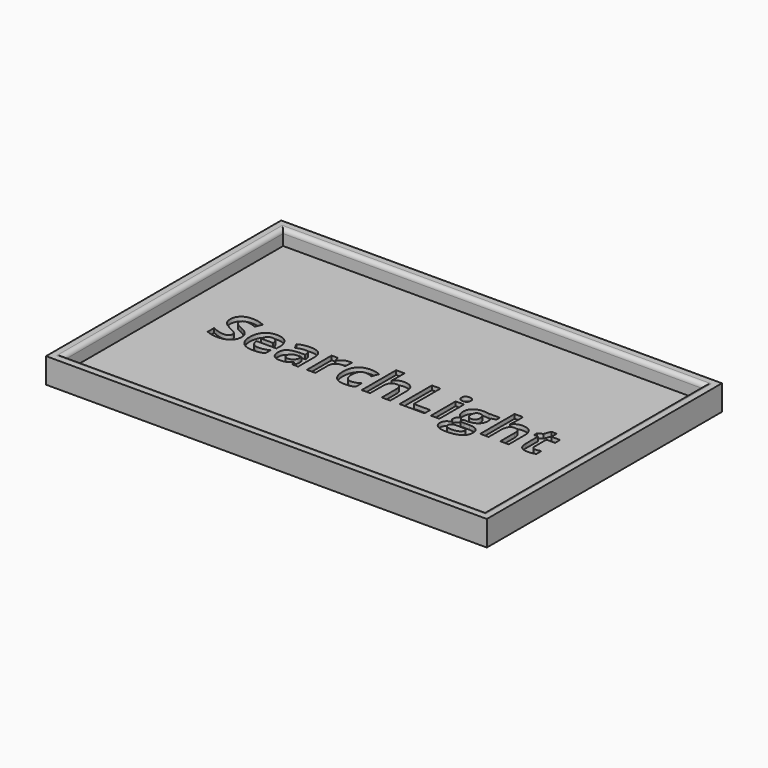
from build123d import *

# Parameters (mm, degrees)
F0_W         = 105
F0_H         = 70
F1_DEPTH     = 6
F2_T         = -2.4
F3_T1_DEPTH  = 65.2
F3_T3_DEPTH  = 100.2
F3_T9_DEPTH  = 67.7
F3_T14_DEPTH = 102.7
F3_T22_DEPTH = 67.7
F3_T27_DEPTH = 102.7
F3_T35_DEPTH = 102.7
F3_T40_DEPTH = 67.7
F3_T48_DEPTH = 67.7
F3_T53_DEPTH = 102.7
F4_TEXT_SIZE = 13.4903696677
F5_DEPTH     = 1


# Not quite as in the source:
# - a fillet or chamfer that OpenCascade refuses, or shapes differently, is made with other operations: its cross-section is extruded or revolved along the edge and cut away or added
# - Text() gives the source's letters only with a copy of the font that has no kerning and outlines rounded to 1/6400 em; it was checked with that copy


with BuildPart() as f1:
    # F0 (on Top) → F1 (new body)
    with BuildSketch(Plane.XY):
        with Locations((52.5, 35)):
            Rectangle(F0_W, F0_H)
    extrude(amount=F1_DEPTH)

    # F2
    f2_openings = [f1.faces().sort_by_distance(p)[0] for p in [
        (52.5, 35, 6),
    ]]
    offset(amount=F2_T, openings=f2_openings)

    # F3: fillet of radius 1 on 8 edges, made by hand

    # F3_s2 → F3_t1 (cut)
    with BuildSketch(Plane.XZ.offset(-67.6)):
        with BuildLine():
            ThreePointArc((1.4, 6), (2.1071067812, 5.7071067812), (2.4, 5))
            Line((2.4, 5), (2.4, 6))
            Line((2.4, 6), (1.4, 6))
        make_face()
        with BuildLine():
            ThreePointArc((103.6, 6), (102.8928932188, 5.7071067812), (102.6, 5))
            Line((102.6, 5), (102.6, 6))
            Line((102.6, 6), (103.6, 6))
        make_face()
    extrude(amount=F3_T1_DEPTH, mode=Mode.SUBTRACT)

    # F3_s4 → F3_t3 (cut)
    with BuildSketch(Plane.YZ.offset(2.4)):
        with BuildLine():
            ThreePointArc((68.6, 6), (67.8928932188, 5.7071067812), (67.6, 5))
            Line((67.6, 5), (67.6, 6))
            Line((67.6, 6), (68.6, 6))
        make_face()
        with BuildLine():
            ThreePointArc((1.4, 6), (2.1071067812, 5.7071067812), (2.4, 5))
            Line((2.4, 5), (2.4, 6))
            Line((2.4, 6), (1.4, 6))
        make_face()
    extrude(amount=F3_T3_DEPTH, mode=Mode.SUBTRACT)


with BuildPart() as f3_tool7:
    # F3_s8 → F3_t9 (new body)
    with BuildSketch(Plane.XZ.offset(-70.1)):
        with BuildLine():
            ThreePointArc((1.4, 6), (2.1071067812, 5.7071067812), (2.4, 5))
            Line((2.4, 5), (2.4, 6))
            Line((2.4, 6), (1.4, 6))
        make_face()
    extrude(amount=F3_T9_DEPTH)

    split(bisect_by=Plane.XZ.offset(-70), keep=Keep.TOP)

    split(bisect_by=Plane.XZ.offset(-67.6), keep=Keep.BOTTOM)


with BuildPart() as f3_tool12:
    # F3_s13 → F3_t14 (new body)
    with BuildSketch(Plane.YZ.offset(102.6)):
        with BuildLine():
            ThreePointArc((68.6, 6), (67.8928932188, 5.7071067812), (67.6, 5))
            Line((67.6, 5), (67.6, 6))
            Line((67.6, 6), (68.6, 6))
        make_face()
    extrude(amount=-F3_T14_DEPTH)

    split(bisect_by=Plane.YZ, keep=Keep.TOP)

    split(bisect_by=Plane.YZ.offset(2.4), keep=Keep.BOTTOM)


with BuildPart() as f3_tool7_1:
    add(f3_tool7.part)

    # F3_t17: intersect F3_tool12
    add(f3_tool12.part, mode=Mode.INTERSECT)


with BuildPart() as f1_1:
    add(f1.part)

    # F3_t5: cut F3_tool7
    add(f3_tool7_1.part, mode=Mode.SUBTRACT)


with BuildPart() as f3_tool20:
    # F3_s21 → F3_t22 (new body)
    with BuildSketch(Plane.XZ.offset(-67.6)):
        with BuildLine():
            ThreePointArc((1.4, 6), (2.1071067812, 5.7071067812), (2.4, 5))
            Line((2.4, 5), (2.4, 6))
            Line((2.4, 6), (1.4, 6))
        make_face()
    extrude(amount=F3_T22_DEPTH)

    split(bisect_by=Plane.XZ, keep=Keep.BOTTOM)

    split(bisect_by=Plane.XZ.offset(-2.4), keep=Keep.TOP)


with BuildPart() as f3_tool25:
    # F3_s26 → F3_t27 (new body)
    with BuildSketch(Plane.YZ.offset(-0.1)):
        with BuildLine():
            ThreePointArc((1.4, 6), (2.1071067812, 5.7071067812), (2.4, 5))
            Line((2.4, 5), (2.4, 6))
            Line((2.4, 6), (1.4, 6))
        make_face()
    extrude(amount=F3_T27_DEPTH)

    split(bisect_by=Plane.YZ, keep=Keep.TOP)

    split(bisect_by=Plane.YZ.offset(2.4), keep=Keep.BOTTOM)


with BuildPart() as f3_tool20_1:
    add(f3_tool20.part)

    # F3_t30: intersect F3_tool25
    add(f3_tool25.part, mode=Mode.INTERSECT)


with BuildPart() as f1_2:
    add(f1_1.part)

    # F3_t18: cut F3_tool20
    add(f3_tool20_1.part, mode=Mode.SUBTRACT)


with BuildPart() as f3_tool33:
    # F3_s34 → F3_t35 (new body)
    with BuildSketch(Plane.YZ.offset(105.1)):
        with BuildLine():
            ThreePointArc((68.6, 6), (67.8928932188, 5.7071067812), (67.6, 5))
            Line((67.6, 5), (67.6, 6))
            Line((67.6, 6), (68.6, 6))
        make_face()
    extrude(amount=-F3_T35_DEPTH)

    split(bisect_by=Plane.YZ.offset(105), keep=Keep.BOTTOM)

    split(bisect_by=Plane.YZ.offset(102.6), keep=Keep.TOP)


with BuildPart() as f3_tool38:
    # F3_s39 → F3_t40 (new body)
    with BuildSketch(Plane.XZ.offset(-2.4)):
        with BuildLine():
            ThreePointArc((103.6, 6), (102.8928932188, 5.7071067812), (102.6, 5))
            Line((102.6, 5), (102.6, 6))
            Line((102.6, 6), (103.6, 6))
        make_face()
    extrude(amount=-F3_T40_DEPTH)

    split(bisect_by=Plane.XZ.offset(-70), keep=Keep.TOP)

    split(bisect_by=Plane.XZ.offset(-67.6), keep=Keep.BOTTOM)


with BuildPart() as f3_tool33_1:
    add(f3_tool33.part)

    # F3_t43: intersect F3_tool38
    add(f3_tool38.part, mode=Mode.INTERSECT)


with BuildPart() as f1_3:
    add(f1_2.part)

    # F3_t31: cut F3_tool33
    add(f3_tool33_1.part, mode=Mode.SUBTRACT)


with BuildPart() as f3_tool46:
    # F3_s47 → F3_t48 (new body)
    with BuildSketch(Plane.XZ.offset(0.1)):
        with BuildLine():
            ThreePointArc((103.6, 6), (102.8928932188, 5.7071067812), (102.6, 5))
            Line((102.6, 5), (102.6, 6))
            Line((102.6, 6), (103.6, 6))
        make_face()
    extrude(amount=-F3_T48_DEPTH)

    split(bisect_by=Plane.XZ, keep=Keep.BOTTOM)

    split(bisect_by=Plane.XZ.offset(-2.4), keep=Keep.TOP)


with BuildPart() as f3_tool51:
    # F3_s52 → F3_t53 (new body)
    with BuildSketch(Plane.YZ.offset(2.4)):
        with BuildLine():
            ThreePointArc((1.4, 6), (2.1071067812, 5.7071067812), (2.4, 5))
            Line((2.4, 5), (2.4, 6))
            Line((2.4, 6), (1.4, 6))
        make_face()
    extrude(amount=F3_T53_DEPTH)

    split(bisect_by=Plane.YZ.offset(105), keep=Keep.BOTTOM)

    split(bisect_by=Plane.YZ.offset(102.6), keep=Keep.TOP)


with BuildPart() as f3_tool46_1:
    add(f3_tool46.part)

    # F3_t56: intersect F3_tool51
    add(f3_tool51.part, mode=Mode.INTERSECT)


with BuildPart() as f1_4:
    add(f1_3.part)

    # F3_t44: cut F3_tool46
    add(f3_tool46_1.part, mode=Mode.SUBTRACT)

    # F4 (on face) → F5 (cut)
    with BuildSketch(Plane.XY.offset(2.4)):
        with Locations((12.4, 31.4)):
            Text('SearchLight', F4_TEXT_SIZE, font='Open Sans', font_style=FontStyle.BOLD, text_align=(TextAlign.LEFT, TextAlign.BOTTOM))
    extrude(amount=-F5_DEPTH, mode=Mode.SUBTRACT)


solid = f1_4.part
